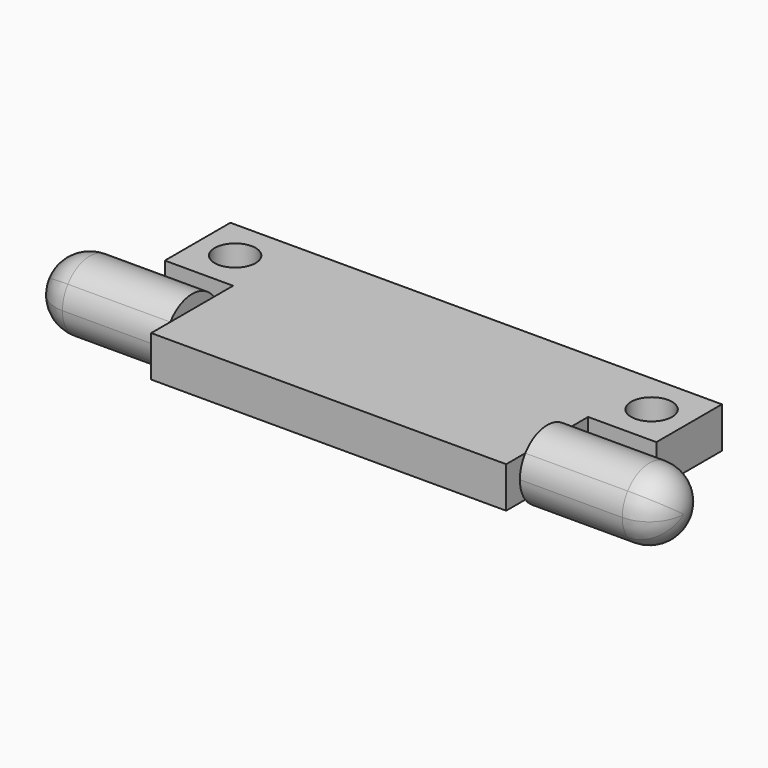
from build123d import *

# Parameters (mm, degrees)
F0_R     = 1.5
F1_DEPTH = 3
F3_DEPTH = 10
F4_R     = 2.5


# Not quite as in the source:
# - a pattern or mirror of a feature is missing from the dataset's text; its kind, count and spacing are read off the source's solid


with BuildPart() as f1:
    # F0 (on Top) → F1 (new body)
    with BuildSketch(Plane.XY):
        Polygon((18, 0.75), (18, 6.75), (-18, 6.75), (-18, 0.75), (-13, 0.75), (-13, -6.75), (13, -6.75), (13, 0.75), align=None)
        with Locations((-15.25, 3.75)):
            Circle(F0_R, mode=Mode.SUBTRACT)
        with Locations((15.25, 3.75)):
            Circle(F0_R, mode=Mode.SUBTRACT)
    extrude(amount=F1_DEPTH)

    # F2 (on face) → F3 (join)
    with BuildSketch(Plane(origin=(-13, 0, 0), x_dir=(0, -1, 0), z_dir=(-1, 0, 0))):
        with BuildLine():
            ThreePointArc((1, 0), (3, -1), (5, 0))
            Line((5, 0), (1, 0))
        make_face()
        with BuildLine():
            ThreePointArc((5, 0), (5.3717082451, 0.709430585), (5.5, 1.5))
            ThreePointArc((5.5, 1.5), (5.3717082451, 2.290569415), (5, 3))
            Line((5, 3), (1, 3))
            ThreePointArc((1, 3), (0.5, 1.5), (1, 0))
            Line((1, 0), (5, 0))
        make_face()
        with BuildLine():
            Line((1, 3), (5, 3))
            ThreePointArc((5, 3), (3, 4), (1, 3))
        make_face()
    f3 = extrude(amount=F3_DEPTH)

    # F3_copies: F3 across plane
    add(f3.mirror(Plane(origin=(0, 0, 0), x_dir=(0, 0, 1), z_dir=(1, 0, 0))))

    # F4
    f4_edges = [f1.edges().sort_by_distance(p)[0] for p in [
        (-23, -1, 0),
        (23, -1, 0),
    ]]
    fillet(f4_edges, radius=F4_R)


solid = f1.part
